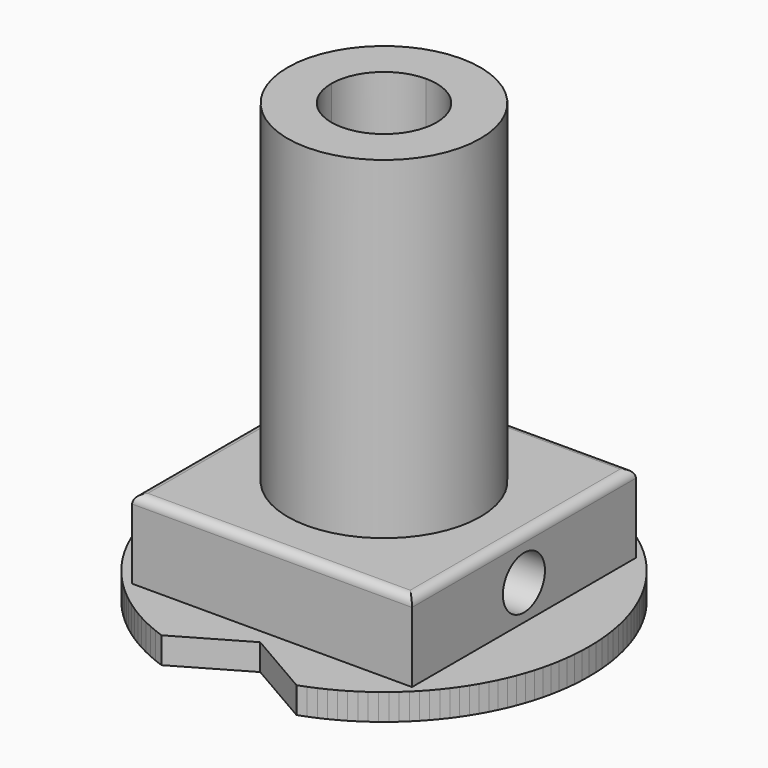
from build123d import *

# Parameters (mm, degrees)
F0_W     = 15.97
F0_H     = 15.97
F1_DEPTH = 1.5
F2_DEPTH = 6
F3_DEPTH = 14
F4_R     = 0.5
F5_DEPTH = 25
F7_D     = 3


# Not quite as in the source:
# - after a boolean that leaves OpenCascade's solid faulty, fix() repairs it


with BuildPart() as f1:
    # F0 (on Top) → F1 (new body)
    with BuildSketch(Plane.XY):
        Polygon((11.463976, 2.379747), (11.359373, 2.838321), (11.236939, 3.290208), (11.097035, 3.735011), (10.940019, 4.172325), (10.766249, 4.60174), (10.576084, 5.022839), (10.369884, 5.435203), (10.148011, 5.838407), (9.910829, 6.232024), (9.658704, 6.615624), (9.392003, 6.988776), (9.111097, 7.351047), (8.816357, 7.702006), (8.508156, 8.04122), (8.186868, 8.368258), (7.852869, 8.68269), (7.506532, 8.98409), (7.148231, 9.272031), (6.778339, 9.546091), (6.397225, 9.805849), (6.005257, 10.050886), (5.602798, 10.280786), (5.190206, 10.495134), (4.767834, 10.693518), (4.336029, 10.875525), (3.895133, 11.040743), (3.851403, 11.055137), (-0.000321, 8.82993), (-3.850041, 11.056837), (-3.888073, 11.04433), (-4.324324, 10.88112), (-4.752184, 10.701192), (-5.171268, 10.504934), (-5.581182, 10.292736), (-5.98153, 10.06499), (-6.371909, 9.822089), (-6.751914, 9.564429), (-7.121137, 9.292409), (-7.47917, 9.00643), (-7.825602, 8.706896), (-8.160021, 8.394212), (-8.482018, 8.068787), (-8.791184, 7.73103), (-9.087111, 7.38135), (-9.369393, 7.020158), (-9.637626, 6.647865), (-9.89141, 6.26488), (-10.130347, 5.871608), (-10.354039, 5.468455), (-10.562095, 5.055822), (-10.754123, 4.634103), (-10.929732, 4.203692), (-11.088533, 3.764972), (-11.230138, 3.318323), (-11.354158, 2.864116), (-11.4602, 2.402716), (-11.54787, 1.934479), (-11.616771, 1.459754), (-11.666499, 0.978883), (-11.696643, 0.4922), (-11.706789, -8e-05), (-11.696889, -0.484214), (-11.667434, -0.963844), (-11.618789, -1.43855), (-11.551313, -1.907948), (-11.465359, -2.371647), (-11.36128, -2.829248), (-11.239422, -3.280348), (-11.100133, -3.724535), (-10.943759, -4.161393), (-10.770647, -4.590499), (-10.581144, -5.011426), (-10.375599, -5.423743), (-10.154362, -5.827016), (-9.917785, -6.220806), (-9.666223, -6.604675), (-9.400031, -6.978182), (-9.119567, -7.340886), (-8.825191, -7.692347), (-8.517263, -8.032124), (-8.196144, -8.359779), (-7.862195, -8.674874), (-7.515776, -8.976975), (-7.157247, -9.265648), (-6.786965, -9.540464), (-6.405285, -9.800995), (-6.012557, -10.046813), (-5.609128, -10.277496), (-5.195341, -10.492621), (-4.771529, -10.691767), (-4.338024, -10.874511), (-3.895147, -11.040433), (-3.849233, -11.055538), (0.000108, -8.829807), (3.850042, -11.056838), (3.888074, -11.04433), (4.324324, -10.881121), (4.752185, -10.701192), (5.171269, -10.504935), (5.581183, -10.292737), (5.98153, -10.064991), (6.371909, -9.822089), (6.751914, -9.56443), (7.121138, -9.29241), (7.479171, -9.006431), (7.825602, -8.706896), (8.160022, -8.394213), (8.482019, -8.068788), (8.791185, -7.73103), (9.087111, -7.38135), (9.369393, -7.020159), (9.637626, -6.647866), (9.891411, -6.26488), (10.130347, -5.871609), (10.35404, -5.468456), (10.562096, -5.055822), (10.754123, -4.634104), (10.929732, -4.203692), (11.088534, -3.764973), (11.230139, -3.318324), (11.354158, -2.864117), (11.4602, -2.402716), (11.547871, -1.934479), (11.616772, -1.459754), (11.666499, -0.978883), (11.696644, -0.492201), (11.706789, 5.7e-05), (11.696823, 0.486311), (11.667183, 0.967786), (11.618247, 1.444099), (11.550389, 1.914878), align=None)
        Rectangle(F0_W, F0_H, mode=Mode.SUBTRACT)
    extrude(amount=F1_DEPTH)

    # F0 (on Top) → F2 (join)
    with BuildSketch(Plane.XY):
        Rectangle(F0_W, F0_H)
        with BuildLine():
            ThreePointArc((-5.5, 0), (-3.8890872965, 3.8890872965), (0, 5.5))
            ThreePointArc((0, 5.5), (3.8890872965, 3.8890872965), (5.5, 0))
            ThreePointArc((5.5, 0), (3.8890872965, -3.8890872965), (0, -5.5))
            ThreePointArc((0, -5.5), (-3.8890872965, -3.8890872965), (-5.5, 0))
        make_face(mode=Mode.SUBTRACT)
    extrude(amount=F2_DEPTH)

    # F0 (on Top) → F3 (join)
    with BuildSketch(Plane.XY):
        with BuildLine():
            ThreePointArc((5.5, 0), (3.8890872965, 3.8890872965), (0, 5.5))
            ThreePointArc((0, 5.5), (-3.8890872965, 3.8890872965), (-5.5, 0))
            ThreePointArc((-5.5, 0), (-3.8890872965, -3.8890872965), (0, -5.5))
            ThreePointArc((0, -5.5), (3.8890872965, -3.8890872965), (5.5, 0))
        make_face()
        with BuildLine():
            ThreePointArc((-3, 0), (-2.1213203436, 2.1213203436), (0, 3))
            ThreePointArc((0, 3), (2.1213203436, 2.1213203436), (3, 0))
            ThreePointArc((3, 0), (2.1213203436, -2.1213203436), (0, -3))
            ThreePointArc((0, -3), (-2.1213203436, -2.1213203436), (-3, 0))
        make_face(mode=Mode.SUBTRACT)
    extrude(amount=F3_DEPTH)

    # F4
    f4_edges = [f1.edges().sort_by_distance(p)[0] for p in [
        (-7.985, 0, 6),
        (0, -7.985, 6),
        (7.985, 0, 6),
        (0, 7.985, 6),
    ]]
    fillet(f4_edges, radius=F4_R)

    # F0 (on Top) → F5 (join)
    with BuildSketch(Plane.XY):
        with BuildLine():
            ThreePointArc((5.5, 0), (3.8890872965, 3.8890872965), (0, 5.5))
            ThreePointArc((0, 5.5), (-3.8890872965, 3.8890872965), (-5.5, 0))
            ThreePointArc((-5.5, 0), (-3.8890872965, -3.8890872965), (0, -5.5))
            ThreePointArc((0, -5.5), (3.8890872965, -3.8890872965), (5.5, 0))
        make_face()
        with BuildLine():
            ThreePointArc((-3, 0), (-2.1213203436, 2.1213203436), (0, 3))
            ThreePointArc((0, 3), (2.1213203436, 2.1213203436), (3, 0))
            ThreePointArc((3, 0), (2.1213203436, -2.1213203436), (0, -3))
            ThreePointArc((0, -3), (-2.1213203436, -2.1213203436), (-3, 0))
        make_face(mode=Mode.SUBTRACT)
    extrude(amount=F5_DEPTH)

    # F7 (through all)
    with Locations(Plane(origin=(-7.985, 0, 0), x_dir=(0, -1, 0), z_dir=(-1, 0, 0))):
        with Locations((0, 3.5)):
            Hole(F7_D / 2)

    add(f1.part.fix(), mode=Mode.REPLACE)


solid = f1.part
